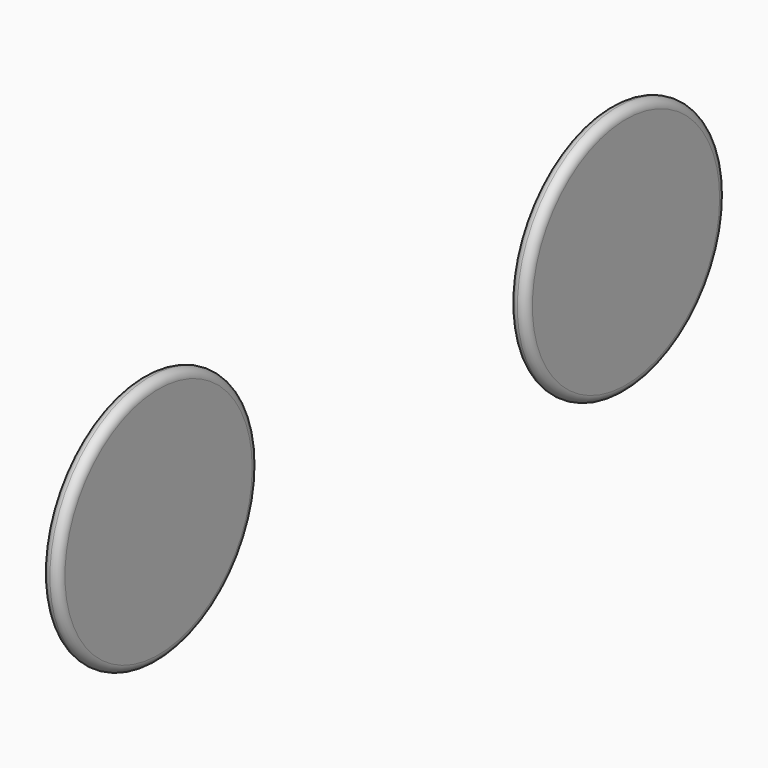
from build123d import *

# Parameters (mm, degrees)
F0_R     = 19.05
F1_DEPTH = 1.27
F2_R     = 1.26999
F2_2_R   = 1.26999


# Not quite as in the source:
# - a fillet or chamfer is up to 0.001 mm smaller than in the source, because OpenCascade refuses the exact size


with BuildPart() as f1:
    # F0 (on Right) → F1 (new body, symmetric)
    with BuildSketch(Plane.YZ):
        with Locations((-88.7891860319, 0)):
            Circle(F0_R)
    extrude(amount=F1_DEPTH, both=True)

    # F2#2 (radius 1.27 in the source; OpenCascade refuses exactly that, so slightly less here)
    f2_2_edges = [f1.edges().sort_by_distance(p)[0] for p in [
        (1.27, -107.839186, 0),
        (-1.27, -107.839186, 0),
    ]]
    fillet(f2_2_edges, radius=F2_2_R)


with BuildPart() as f1b:
    # F0 (on Right) → F1, piece 2 (new body, symmetric)
    with BuildSketch(Plane.YZ):
        Circle(F0_R)
    extrude(amount=F1_DEPTH, both=True)

    # F2 (radius 1.27 in the source; OpenCascade refuses exactly that, so slightly less here)
    f2_edges = [f1b.edges().sort_by_distance(p)[0] for p in [
        (1.27, -19.05, 0),
        (-1.27, -19.05, 0),
    ]]
    fillet(f2_edges, radius=F2_R)


solid = Compound([f1.part, f1b.part])
